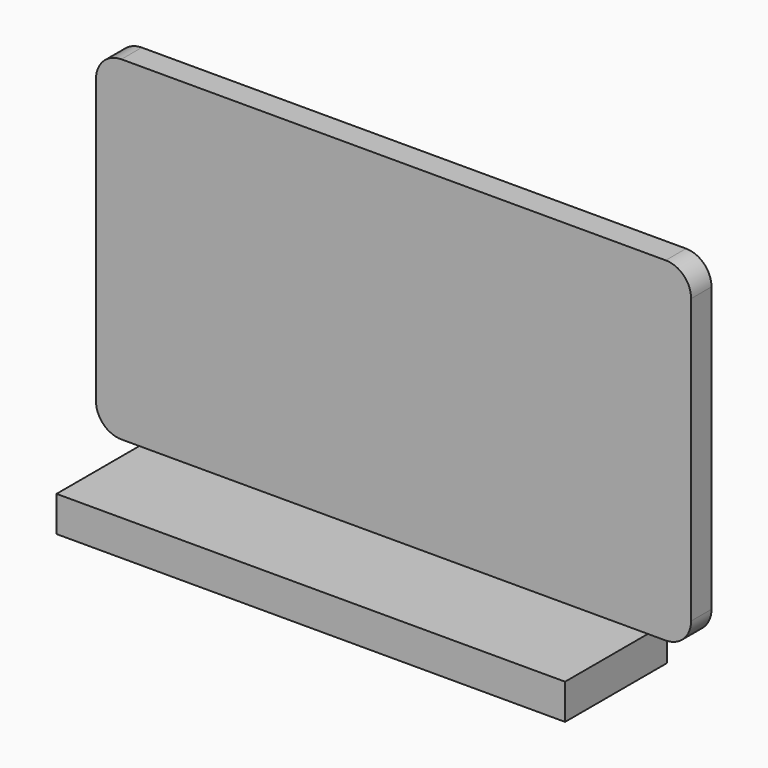
from build123d import *

# Parameters (mm, degrees)
F0_W        = 118.8959814608
F0_H        = 66.8615028262
F1_DEPTH    = 5.08
F2_R        = 5.08
F3_W        = 101.6
F3_H        = 7.0752100054
F4_DEPTH    = 25.4
F5_R        = 5.08
F6_T1_DEPTH = 127
F6_T3_DEPTH = 14.6952100054
F6_T5_DEPTH = 33.02
F6_T8_ANGLE = 90
F7_DEPTH    = 25.4


# Not quite as in the source:
# - a fillet or chamfer that OpenCascade refuses, or shapes differently, is made with other operations: its cross-section is extruded or revolved along the edge and cut away or added


with BuildPart() as f1:
    # F0 (on Front) → F1 (new body)
    with BuildSketch(Plane.XZ):
        with Locations((0.2797562629, 8.6724124849)):
            Rectangle(F0_W, F0_H)
    extrude(amount=F1_DEPTH)

    # F2
    f2_edges = [f1.edges().sort_by_distance(p)[0] for p in [
        (59.727747, -2.54, 42.103164),
        (-59.168234, -2.54, 42.103164),
        (-59.168234, -2.54, -24.758339),
        (59.727747, -2.54, -24.758339),
    ]]
    fillet(f2_edges, radius=F2_R)


with BuildPart() as f4:
    # F3 (on Front) → F4 (new body)
    with BuildSketch(Plane.XZ):
        with Locations((0, -28.5350345075)):
            Rectangle(F3_W, F3_H)
    extrude(amount=F4_DEPTH)

    # F5
    f5_edges = [f4.edges().sort_by_distance(p)[0] for p in [
        (0, -25.4, -32.07264),
    ]]
    fillet(f5_edges, radius=F5_R)

    # F6: fillet of radius 5.08 on 3 edges, made by hand

    # F6_s2 → F6_t1 (cut)
    with BuildSketch(Plane.YZ.offset(-63.5)):
        with BuildLine():
            ThreePointArc((-5.08, -32.0726395102), (-1.4878975516, -30.5847419586), (0, -26.9926395102))
            Line((0, -26.9926395102), (0, -32.0726395102))
            Line((0, -32.0726395102), (-5.08, -32.0726395102))
        make_face()
        with BuildLine():
            ThreePointArc((-25.4, -30.0774295048), (-23.9121024484, -26.4853270564), (-20.32, -24.9974295048))
            Line((-20.32, -24.9974295048), (-25.4, -24.9974295048))
            Line((-25.4, -24.9974295048), (-25.4, -30.0774295048))
        make_face()
    extrude(amount=F6_T1_DEPTH, mode=Mode.SUBTRACT)

    # F6_s4 → F6_t3 (cut)
    with BuildSketch(Plane.XY.offset(-26.9926395102)):
        with BuildLine():
            ThreePointArc((-45.72, -25.4), (-49.3121024484, -23.9121024484), (-50.8, -20.32))
            Line((-50.8, -20.32), (-50.8, -25.4))
            Line((-50.8, -25.4), (-45.72, -25.4))
        make_face()
    extrude(amount=F6_T3_DEPTH, mode=Mode.SUBTRACT)

    # F6_s6 → F6_t5 (cut)
    with BuildSketch(Plane.XZ.offset(-12.7)):
        with BuildLine():
            ThreePointArc((-45.72, -32.0726395102), (-49.3121024484, -30.5847419586), (-50.8, -26.9926395102))
            Line((-50.8, -26.9926395102), (-50.8, -32.0726395102))
            Line((-50.8, -32.0726395102), (-45.72, -32.0726395102))
        make_face()
    extrude(amount=F6_T5_DEPTH, mode=Mode.SUBTRACT)

    # F6_s7 → F6_t8 (revolve, cut)
    with BuildSketch(Plane.XZ.offset(20.32)):
        with BuildLine():
            ThreePointArc((-45.72, -32.0726395102), (-49.3121024484, -30.5847419586), (-50.8, -26.9926395102))
            Line((-50.8, -26.9926395102), (-50.8, -32.0726395102))
            Line((-50.8, -32.0726395102), (-45.72, -32.0726395102))
        make_face()
    revolve(axis=Axis((-50.8, -20.32, -26.9926395102), (-1, 0, 0)), revolution_arc=F6_T8_ANGLE, mode=Mode.SUBTRACT)

    # F3 (on Front) → F7 (join)
    with BuildSketch(Plane.XZ):
        with Locations((0, -28.5350345075)):
            Rectangle(F3_W, F3_H)
    extrude(amount=F7_DEPTH)


solid = Compound([f1.part, f4.part])
